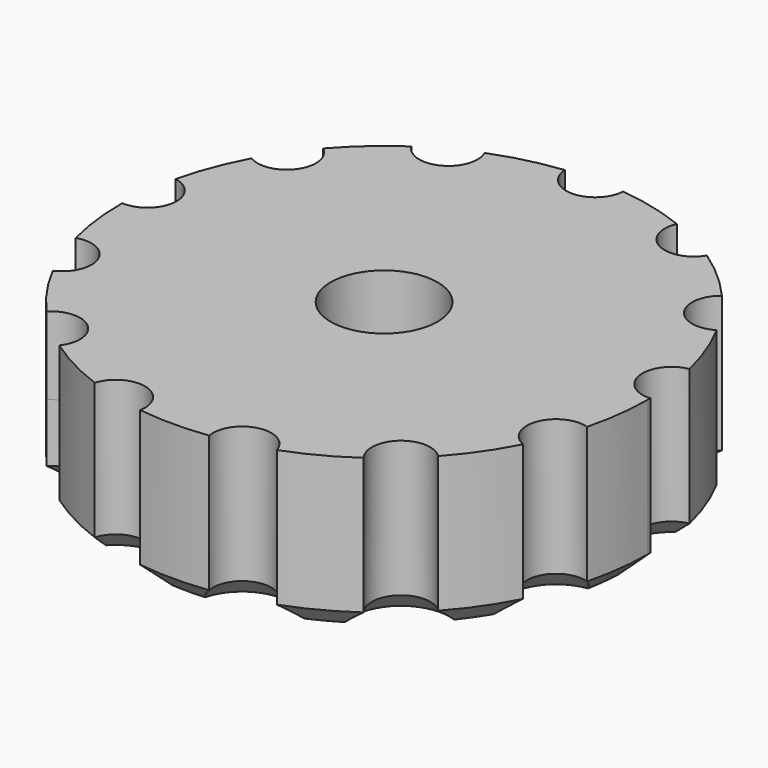
from build123d import *

# Parameters (mm, degrees)
F0_R         = 9
F0_R_2       = 2.75
F1_DEPTH     = 4
F2_DEPTH     = 4
F3_T2_ANGLE  = 36.7292460902
F3_T4_ANGLE  = 359.64
F3_T6_ANGLE  = 36.7292460902
F3_T8_ANGLE  = 359.64
F3_T10_ANGLE = 36.7292460902
F3_T12_ANGLE = 359.64
F3_T14_ANGLE = 36.7292460902
F3_T16_ANGLE = 359.64
F3_T18_ANGLE = 36.7292460902
F3_T20_ANGLE = 359.64
F3_T22_ANGLE = 36.7292460902
F3_T24_ANGLE = 359.64
F3_T26_ANGLE = 36.7292460902
F3_T28_ANGLE = 359.64
F3_T30_ANGLE = 36.7292460902
F3_T32_ANGLE = 359.64
F3_T34_ANGLE = 36.7292460902
F3_T36_ANGLE = 359.64
F3_T38_ANGLE = 36.7292460902
F3_T40_ANGLE = 359.64
F3_T42_ANGLE = 36.7292460902
F3_T44_ANGLE = 359.64
F3_T46_ANGLE = 36.7292460902
F3_T48_ANGLE = 359.64
F3_T50_ANGLE = 36.7292460902
F3_T52_ANGLE = 359.64


# Not quite as in the source:
# - a fillet or chamfer that OpenCascade refuses, or shapes differently, is made with other operations: its cross-section is extruded or revolved along the edge and cut away or added


with BuildPart() as f1:
    # F0 (on Top) → F1 (new body)
    with BuildSketch(Plane.XY):
        with BuildLine():
            ThreePointArc((13.1511570809, -3.3857742739), (13.4723626948, -1.7064124416), (13.58, 0))
            ThreePointArc((13.58, 0), (13.579819293, 0.0700568992), (13.5792771769, 0.1401119339))
            ThreePointArc((13.5792771769, 0.1401119339), (11.9919231991, 1.4560830975), (13.218219042, 3.1136932024))
            ThreePointArc((13.218219042, 3.1136932024), (12.6975205757, 4.815534366), (11.9587395379, 6.4346677198))
            ThreePointArc((11.9587395379, 6.4346677198), (9.9416451, 6.8622221405), (10.2571463173, 8.89985109))
            ThreePointArc((10.2571463173, 8.89985109), (9.0052056989, 10.1647759602), (7.5985987892, 11.2551186773))
            ThreePointArc((7.5985987892, 11.2551186773), (5.6138559183, 10.6963087899), (4.9462849834, 12.6471603478))
            ThreePointArc((4.9462849834, 12.6471603478), (3.249906721, 13.1853898806), (1.497710631, 13.4971575847))
            ThreePointArc((1.497710631, 13.4971575847), (0, 12.08), (-1.497710631, 13.4971575847))
            ThreePointArc((-1.497710631, 13.4971575847), (-3.249906721, 13.1853898806), (-4.9462849834, 12.6471603478))
            ThreePointArc((-4.9462849834, 12.6471603478), (-4.845167239, 12.3430963913), (-4.8109406764, 12.0244928284))
            ThreePointArc((-4.8109406764, 12.0244928284), (-5.9118712396, 10.5785524476), (-7.5985987892, 11.2551186773))
            ThreePointArc((-7.5985987892, 11.2551186773), (-9.0052056989, 10.1647759602), (-10.2571463173, 8.89985109))
            ThreePointArc((-10.2571463173, 8.89985109), (-9.8291869969, 8.3744473269), (-9.6761208988, 7.7143192606))
            ThreePointArc((-9.6761208988, 7.7143192606), (-10.4426115119, 6.4058988468), (-11.9587395379, 6.4346677198))
            ThreePointArc((-11.9587395379, 6.4346677198), (-12.6975205757, 4.815534366), (-13.218219042, 3.1136932024))
            ThreePointArc((-13.218219042, 3.1136932024), (-12.3311710463, 2.6001764438), (-11.9809865103, 1.6368881179))
            ThreePointArc((-11.9809865103, 1.6368881179), (-12.4556660725, 0.5420283095), (-13.5792771769, 0.1401119339))
            ThreePointArc((-13.5792771769, 0.1401119339), (-13.4809865103, -1.6368881179), (-13.1511570809, -3.3857742739))
            ThreePointArc((-13.1511570809, -3.3857742739), (-11.811646645, -3.6050685966), (-11.1975205757, -4.815534366))
            ThreePointArc((-11.1975205757, -4.815534366), (-11.4399769841, -5.6332042965), (-12.0889660626, -6.1865418075))
            ThreePointArc((-12.0889660626, -6.1865418075), (-11.1761208988, -7.7143192606), (-10.0713235212, -9.109601667))
            ThreePointArc((-10.0713235212, -9.109601667), (-8.4347570743, -8.7774806179), (-7.5052056989, -10.1647759602))
            ThreePointArc((-7.5052056989, -10.1647759602), (-7.588522816, -10.6577360085), (-7.8292185113, -11.0959333768))
            ThreePointArc((-7.8292185113, -11.0959333768), (-6.3109406764, -12.0244928284), (-4.6842711154, -12.7465291008))
            ThreePointArc((-4.6842711154, -12.7465291008), (-3.0280358031, -11.7018895282), (-1.749906721, -13.1853898806))
            ThreePointArc((-1.749906721, -13.1853898806), (-1.7564170065, -13.3249910007), (-1.7758913513, -13.4633803299))
            ThreePointArc((-1.7758913513, -13.4633803299), (0, -13.58), (1.7758913513, -13.4633803299))
            ThreePointArc((1.7758913513, -13.4633803299), (2.8909332246, -11.7289771545), (4.6842711154, -12.7465291008))
            ThreePointArc((4.6842711154, -12.7465291008), (6.3109406764, -12.0244928284), (7.8292185113, -11.0959333768))
            ThreePointArc((7.8292185113, -11.0959333768), (8.0105217115, -9.0420098379), (10.0713235212, -9.109601667))
            ThreePointArc((10.0713235212, -9.109601667), (11.1761208988, -7.7143192606), (12.0889660626, -6.1865418075))
            ThreePointArc((12.0889660626, -6.1865418075), (11.2949962116, -4.2836270355), (13.1511570809, -3.3857742739))
        make_face()
        Circle(F0_R, mode=Mode.SUBTRACT)
        Circle(F0_R)
        Circle(F0_R_2, mode=Mode.SUBTRACT)
    extrude(amount=F1_DEPTH)

    # F0 (on Top) → F2 (join)
    with BuildSketch(Plane.XY):
        with BuildLine():
            ThreePointArc((13.1511570809, -3.3857742739), (13.4723626948, -1.7064124416), (13.58, 0))
            ThreePointArc((13.58, 0), (13.579819293, 0.0700568992), (13.5792771769, 0.1401119339))
            ThreePointArc((13.5792771769, 0.1401119339), (11.9919231991, 1.4560830975), (13.218219042, 3.1136932024))
            ThreePointArc((13.218219042, 3.1136932024), (12.6975205757, 4.815534366), (11.9587395379, 6.4346677198))
            ThreePointArc((11.9587395379, 6.4346677198), (9.9416451, 6.8622221405), (10.2571463173, 8.89985109))
            ThreePointArc((10.2571463173, 8.89985109), (9.0052056989, 10.1647759602), (7.5985987892, 11.2551186773))
            ThreePointArc((7.5985987892, 11.2551186773), (5.6138559183, 10.6963087899), (4.9462849834, 12.6471603478))
            ThreePointArc((4.9462849834, 12.6471603478), (3.249906721, 13.1853898806), (1.497710631, 13.4971575847))
            ThreePointArc((1.497710631, 13.4971575847), (0, 12.08), (-1.497710631, 13.4971575847))
            ThreePointArc((-1.497710631, 13.4971575847), (-3.249906721, 13.1853898806), (-4.9462849834, 12.6471603478))
            ThreePointArc((-4.9462849834, 12.6471603478), (-4.845167239, 12.3430963913), (-4.8109406764, 12.0244928284))
            ThreePointArc((-4.8109406764, 12.0244928284), (-5.9118712396, 10.5785524476), (-7.5985987892, 11.2551186773))
            ThreePointArc((-7.5985987892, 11.2551186773), (-9.0052056989, 10.1647759602), (-10.2571463173, 8.89985109))
            ThreePointArc((-10.2571463173, 8.89985109), (-9.8291869969, 8.3744473269), (-9.6761208988, 7.7143192606))
            ThreePointArc((-9.6761208988, 7.7143192606), (-10.4426115119, 6.4058988468), (-11.9587395379, 6.4346677198))
            ThreePointArc((-11.9587395379, 6.4346677198), (-12.6975205757, 4.815534366), (-13.218219042, 3.1136932024))
            ThreePointArc((-13.218219042, 3.1136932024), (-12.3311710463, 2.6001764438), (-11.9809865103, 1.6368881179))
            ThreePointArc((-11.9809865103, 1.6368881179), (-12.4556660725, 0.5420283095), (-13.5792771769, 0.1401119339))
            ThreePointArc((-13.5792771769, 0.1401119339), (-13.4809865103, -1.6368881179), (-13.1511570809, -3.3857742739))
            ThreePointArc((-13.1511570809, -3.3857742739), (-11.811646645, -3.6050685966), (-11.1975205757, -4.815534366))
            ThreePointArc((-11.1975205757, -4.815534366), (-11.4399769841, -5.6332042965), (-12.0889660626, -6.1865418075))
            ThreePointArc((-12.0889660626, -6.1865418075), (-11.1761208988, -7.7143192606), (-10.0713235212, -9.109601667))
            ThreePointArc((-10.0713235212, -9.109601667), (-8.4347570743, -8.7774806179), (-7.5052056989, -10.1647759602))
            ThreePointArc((-7.5052056989, -10.1647759602), (-7.588522816, -10.6577360085), (-7.8292185113, -11.0959333768))
            ThreePointArc((-7.8292185113, -11.0959333768), (-6.3109406764, -12.0244928284), (-4.6842711154, -12.7465291008))
            ThreePointArc((-4.6842711154, -12.7465291008), (-3.0280358031, -11.7018895282), (-1.749906721, -13.1853898806))
            ThreePointArc((-1.749906721, -13.1853898806), (-1.7564170065, -13.3249910007), (-1.7758913513, -13.4633803299))
            ThreePointArc((-1.7758913513, -13.4633803299), (0, -13.58), (1.7758913513, -13.4633803299))
            ThreePointArc((1.7758913513, -13.4633803299), (2.8909332246, -11.7289771545), (4.6842711154, -12.7465291008))
            ThreePointArc((4.6842711154, -12.7465291008), (6.3109406764, -12.0244928284), (7.8292185113, -11.0959333768))
            ThreePointArc((7.8292185113, -11.0959333768), (8.0105217115, -9.0420098379), (10.0713235212, -9.109601667))
            ThreePointArc((10.0713235212, -9.109601667), (11.1761208988, -7.7143192606), (12.0889660626, -6.1865418075))
            ThreePointArc((12.0889660626, -6.1865418075), (11.2949962116, -4.2836270355), (13.1511570809, -3.3857742739))
        make_face()
        Circle(F0_R, mode=Mode.SUBTRACT)
    extrude(amount=-F2_DEPTH)

    # F3: chamfer of 1 on 27 edges, made by hand

    # F3_s1 → F3_t2 (revolve, cut)
    with BuildSketch(Plane(origin=(0, 0, 0), x_dir=(0, 0, 1), z_dir=(0.9193151191, 0.3935221873, 0))):
        Polygon((-3, -13.58), (-4, -12.58), (-4, -13.58), align=None)
    revolve(axis=Axis((0, 0, -4), (0, 0, 1)), revolution_arc=F3_T2_ANGLE, mode=Mode.SUBTRACT)

    # F3_s3 → F3_t4 (revolve, cut)
    with BuildSketch(Plane(origin=(-0.0243453928, -0.0350344513, 0), x_dir=(0, 0, 1), z_dir=(-0.5706474193, -0.8211951795, 0))):
        Polygon((-4, 16.0799329854), (-3, 15.0799329854), (-4, 15.0799329854), align=None)
    revolve(axis=Axis((-11.1761208988, 7.7143192606, -4), (0, 0, -1)), revolution_arc=F3_T4_ANGLE, mode=Mode.SUBTRACT)

    # F3_s5 → F3_t6 (revolve, cut)
    with BuildSketch(Plane(origin=(0, 0, 0), x_dir=(0, 0, 1), z_dir=(0.6311342325, 0.7756736302, 0))):
        Polygon((-4, -12.58), (-3, -13.58), (-4, -13.58), align=None)
    revolve(axis=Axis((0, 0, -4), (0, 0, 1)), revolution_arc=F3_T6_ANGLE, mode=Mode.SUBTRACT)

    # F3_s7 → F3_t8 (revolve, cut)
    with BuildSketch(Plane(origin=(-0.0052754534, -0.0423353341, 0), x_dir=(0, 0, 1), z_dir=(-0.1236547672, -0.9923252988, 0))):
        Polygon((-4, 16.0799329854), (-3, 15.0799329854), (-4, 15.0799329854), align=None)
    revolve(axis=Axis((-13.4809865103, 1.6368881179, -4), (0, 0, -1)), revolution_arc=F3_T8_ANGLE, mode=Mode.SUBTRACT)

    # F3_s9 → F3_t10 (revolve, cut)
    with BuildSketch(Plane(origin=(0, 0, 0), x_dir=(0, 0, 1), z_dir=(0.1983680993, 0.9801275923, 0))):
        Polygon((-4, -12.58), (-3, -13.58), (-4, -13.58), align=None)
    revolve(axis=Axis((0, 0, -4), (0, 0, 1)), revolution_arc=F3_T10_ANGLE, mode=Mode.SUBTRACT)

    # F3_s11 → F3_t12 (revolve, cut)
    with BuildSketch(Plane(origin=(0.0150030288, -0.0399377022, 0), x_dir=(0, 0, 1), z_dir=(0.3516657018, -0.9361256508, 0))):
        Polygon((-4, 16.0799329854), (-3, 15.0799329854), (-4, 15.0799329854), align=None)
    revolve(axis=Axis((-12.6975205757, -4.815534366, -4), (0, 0, -1)), revolution_arc=F3_T12_ANGLE, mode=Mode.SUBTRACT)

    # F3_s13 → F3_t14 (revolve, cut)
    with BuildSketch(Plane(origin=(0, 0, 0), x_dir=(0, 0, 1), z_dir=(-0.2798417749, 0.9600461348, 0))):
        Polygon((-4, -12.58), (-3, -13.58), (-4, -13.58), align=None)
    revolve(axis=Axis((0, 0, -4), (0, 0, 1)), revolution_arc=F3_T14_ANGLE, mode=Mode.SUBTRACT)

    # F3_s15 → F3_t16 (revolve, cut)
    with BuildSketch(Plane(origin=(0.0318444978, -0.0283908239, 0), x_dir=(0, 0, 1), z_dir=(0.7464237966, -0.6654708979, 0))):
        Polygon((-4, 16.0799329854), (-3, 15.0799329854), (-4, 15.0799329854), align=None)
    revolve(axis=Axis((-9.0052056989, -10.1647759602, -4), (0, 0, -1)), revolution_arc=F3_T16_ANGLE, mode=Mode.SUBTRACT)

    # F3_s17 → F3_t18 (revolve, cut)
    with BuildSketch(Plane(origin=(0, 0, 0), x_dir=(0, 0, 1), z_dir=(-0.6939432709, 0.7200296777, 0))):
        Polygon((-4, -12.58), (-3, -13.58), (-4, -13.58), align=None)
    revolve(axis=Axis((0, 0, -4), (0, 0, 1)), revolution_arc=F3_T18_ANGLE, mode=Mode.SUBTRACT)

    # F3_s19 → F3_t20 (revolve, cut)
    with BuildSketch(Plane(origin=(0.0413907762, -0.0103399501, 0), x_dir=(0, 0, 1), z_dir=(0.9701851949, -0.242364782, 0))):
        Polygon((-4, 16.0799329854), (-3, 15.0799329854), (-4, 15.0799329854), align=None)
    revolve(axis=Axis((-3.249906721, -13.1853898806, -4), (0, 0, -1)), revolution_arc=F3_T20_ANGLE, mode=Mode.SUBTRACT)

    # F3_s21 → F3_t22 (revolve, cut)
    with BuildSketch(Plane(origin=(0, 0, 0), x_dir=(0, 0, 1), z_dir=(-0.9490707265, 0.3150630987, 0))):
        Polygon((-4, -12.58), (-3, -13.58), (-4, -13.58), align=None)
    revolve(axis=Axis((0, 0, -4), (0, 0, 1)), revolution_arc=F3_T22_ANGLE, mode=Mode.SUBTRACT)

    # F3_s23 → F3_t24 (revolve, cut)
    with BuildSketch(Plane(origin=(0.0414549266, 0.0100796817, 0), x_dir=(0, 0, 1), z_dir=(0.9716888571, 0.2362641846, 0))):
        Polygon((-4, 16.0799329854), (-3, 15.0799329854), (-4, 15.0799329854), align=None)
    revolve(axis=Axis((3.249906721, -13.1853898806, -4), (0, 0, -1)), revolution_arc=F3_T24_ANGLE, mode=Mode.SUBTRACT)

    # F3_s25 → F3_t26 (revolve, cut)
    with BuildSketch(Plane(origin=(0, 0, 0), x_dir=(0, 0, 1), z_dir=(-0.9867775161, -0.1620806393, 0))):
        Polygon((-4, -12.58), (-3, -13.58), (-4, -13.58), align=None)
    revolve(axis=Axis((0, 0, -4), (0, 0, 1)), revolution_arc=F3_T26_ANGLE, mode=Mode.SUBTRACT)

    # F3_s27 → F3_t28 (revolve, cut)
    with BuildSketch(Plane(origin=(0.0320222529, 0.0281901799, 0), x_dir=(0, 0, 1), z_dir=(0.7505903123, 0.6607678739, 0))):
        Polygon((-4, 16.0799329854), (-3, 15.0799329854), (-4, 15.0799329854), align=None)
    revolve(axis=Axis((9.0052056989, -10.1647759602, -4), (0, 0, -1)), revolution_arc=F3_T28_ANGLE, mode=Mode.SUBTRACT)

    # F3_s29 → F3_t30 (revolve, cut)
    with BuildSketch(Plane(origin=(0, 0, 0), x_dir=(0, 0, 1), z_dir=(-0.7984254688, -0.6020936561, 0))):
        Polygon((-4, -12.58), (-3, -13.58), (-4, -13.58), align=None)
    revolve(axis=Axis((0, 0, -4), (0, 0, 1)), revolution_arc=F3_T30_ANGLE, mode=Mode.SUBTRACT)

    # F3_s31 → F3_t32 (revolve, cut)
    with BuildSketch(Plane(origin=(0.0152536669, 0.0398426476, 0), x_dir=(0, 0, 1), z_dir=(0.3575405725, 0.9338976063, 0))):
        Polygon((-4, 16.0799329854), (-3, 15.0799329854), (-4, 15.0799329854), align=None)
    revolve(axis=Axis((12.6975205757, -4.815534366, -4), (0, 0, -1)), revolution_arc=F3_T32_ANGLE, mode=Mode.SUBTRACT)

    # F3_s33 → F3_t34 (revolve, cut)
    with BuildSketch(Plane(origin=(0, 0, 0), x_dir=(0, 0, 1), z_dir=(-0.4271637687, -0.9041742723, 0))):
        Polygon((-4, -12.58), (-3, -13.58), (-4, -13.58), align=None)
    revolve(axis=Axis((0, 0, -4), (0, 0, 1)), revolution_arc=F3_T34_ANGLE, mode=Mode.SUBTRACT)

    # F3_s35 → F3_t36 (revolve, cut)
    with BuildSketch(Plane(origin=(-0.0050093503, 0.0423676449, 0), x_dir=(0, 0, 1), z_dir=(-0.1174174037, 0.9930826518, 0))):
        Polygon((-4, 16.0799329854), (-3, 15.0799329854), (-4, 15.0799329854), align=None)
    revolve(axis=Axis((13.4809865103, 1.6368881179, -4), (0, 0, -1)), revolution_arc=F3_T36_ANGLE, mode=Mode.SUBTRACT)

    # F3_s37 → F3_t38 (revolve, cut)
    with BuildSketch(Plane(origin=(0, 0, 0), x_dir=(0, 0, 1), z_dir=(0.041956003, -0.9991194592, 0))):
        Polygon((-4, -12.58), (-3, -13.58), (-4, -13.58), align=None)
    revolve(axis=Axis((0, 0, -4), (0, 0, 1)), revolution_arc=F3_T38_ANGLE, mode=Mode.SUBTRACT)

    # F3_s39 → F3_t40 (revolve, cut)
    with BuildSketch(Plane(origin=(-0.0241247857, 0.0351867253, 0), x_dir=(0, 0, 1), z_dir=(-0.5654764676, 0.8247644297, 0))):
        Polygon((-4, 16.0799329854), (-3, 15.0799329854), (-4, 15.0799329854), align=None)
    revolve(axis=Axis((11.1761208988, 7.7143192606, -4), (0, 0, -1)), revolution_arc=F3_T40_ANGLE, mode=Mode.SUBTRACT)

    # F3_s41 → F3_t42 (revolve, cut)
    with BuildSketch(Plane(origin=(0, 0, 0), x_dir=(0, 0, 1), z_dir=(0.50146416, -0.8651784187, 0))):
        Polygon((-4, -12.58), (-3, -13.58), (-4, -13.58), align=None)
    revolve(axis=Axis((0, 0, -4), (0, 0, 1)), revolution_arc=F3_T42_ANGLE, mode=Mode.SUBTRACT)

    # F3_s43 → F3_t44 (revolve, cut)
    with BuildSketch(Plane(origin=(-0.0377135235, 0.019944951, 0), x_dir=(0, 0, 1), z_dir=(-0.8839916876, 0.4675026163, 0))):
        Polygon((-4, 16.0799329854), (-3, 15.0799329854), (-4, 15.0799329854), align=None)
    revolve(axis=Axis((6.3109406764, 12.0244928284, -4), (0, 0, -1)), revolution_arc=F3_T44_ANGLE, mode=Mode.SUBTRACT)

    # F3_s45 → F3_t46 (revolve, cut)
    with BuildSketch(Plane(origin=(0, 0, 0), x_dir=(0, 0, 1), z_dir=(0.8460929213, -0.533035429, 0))):
        Polygon((-4, -12.58), (-3, -13.58), (-4, -13.58), align=None)
    revolve(axis=Axis((0, 0, -4), (0, 0, 1)), revolution_arc=F3_T46_ANGLE, mode=Mode.SUBTRACT)

    # F3_s47 → F3_t48 (revolve, cut)
    with BuildSketch(Plane(origin=(-0.0426625475, 0.0001340288, 0), x_dir=(0, 0, 1), z_dir=(-0.9999950652, 0.0031415875, 0))):
        Polygon((-4, 16.0799329854), (-3, 15.0799329854), (-4, 15.0799329854), align=None)
    revolve(axis=Axis((0, 13.58, -4), (0, 0, -1)), revolution_arc=F3_T48_ANGLE, mode=Mode.SUBTRACT)

    # F3_s49 → F3_t50 (revolve, cut)
    with BuildSketch(Plane(origin=(0, 0, 0), x_dir=(0, 0, 1), z_dir=(0.9968919908, -0.0787804463, 0))):
        Polygon((-4, -12.58), (-3, -13.58), (-4, -13.58), align=None)
    revolve(axis=Axis((0, 0, -4), (0, 0, 1)), revolution_arc=F3_T50_ANGLE, mode=Mode.SUBTRACT)

    # F3_s51 → F3_t52 (revolve, cut)
    with BuildSketch(Plane(origin=(-0.0378380961, -0.0197075978, 0), x_dir=(0, 0, 1), z_dir=(-0.8869116246, -0.4619391412, 0))):
        Polygon((-4, 16.0799329854), (-3, 15.0799329854), (-4, 15.0799329854), align=None)
    revolve(axis=Axis((-6.3109406764, 12.0244928284, -4), (0, 0, -1)), revolution_arc=F3_T52_ANGLE, mode=Mode.SUBTRACT)

    # F3_s53 → F3_t54 (revolve, cut)
    with BuildSketch(Plane.XZ):
        Polygon((10, -4), (9, -3), (9, -4), align=None)
    revolve(axis=Axis((0, 0, -4), (0, 0, 1)), mode=Mode.SUBTRACT)


solid = f1.part
